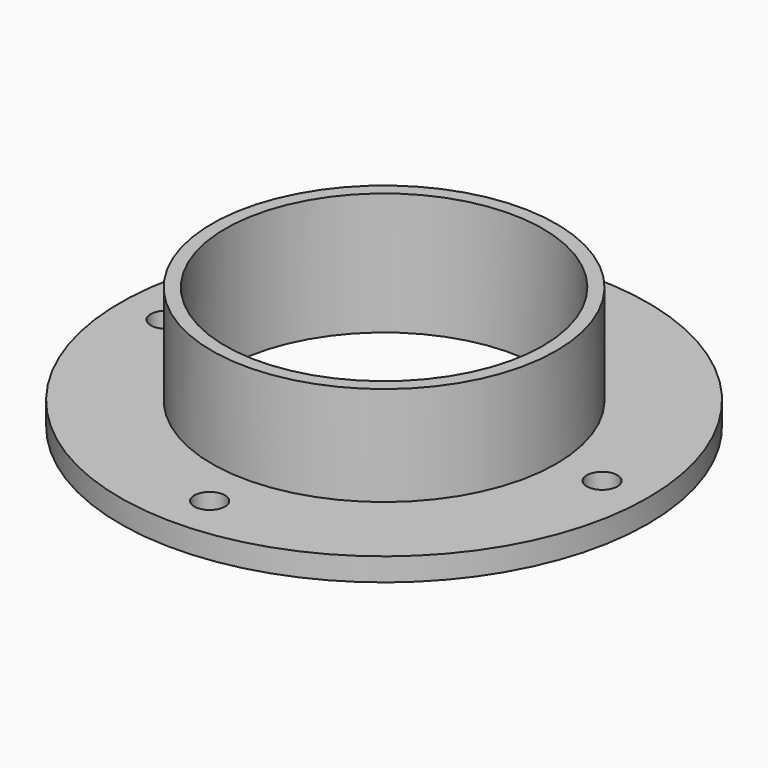
from build123d import *

# Parameters (mm, degrees)
F0_R     = 876.3
F0_R_2   = 50.8
F0_R_3   = 571.5
F1_DEPTH = 76.2
F0_R_4   = 527.05
F2_DEPTH = 406.4


# Not quite as in the source:
# - a feature names something its author has since deleted; it is built from what else it names


with BuildPart() as f1:
    # F0 (on Top) → F1 (new body)
    with BuildSketch(Plane.XY):
        Circle(F0_R)
        with Locations((0, -723.9)):
            Circle(F0_R_2, mode=Mode.SUBTRACT)
        with Locations((-723.9, 0)):
            Circle(F0_R_2, mode=Mode.SUBTRACT)
        Circle(F0_R_3, mode=Mode.SUBTRACT)
        with Locations((723.9, 0)):
            Circle(F0_R_2, mode=Mode.SUBTRACT)
        with Locations((0, 723.9)):
            Circle(F0_R_2, mode=Mode.SUBTRACT)
    extrude(amount=F1_DEPTH)

    # F0 (on Top) → F2 (join)
    with BuildSketch(Plane.XY):
        Circle(F0_R_3)
        Circle(F0_R_4, mode=Mode.SUBTRACT)
    extrude(amount=F2_DEPTH)


solid = f1.part
